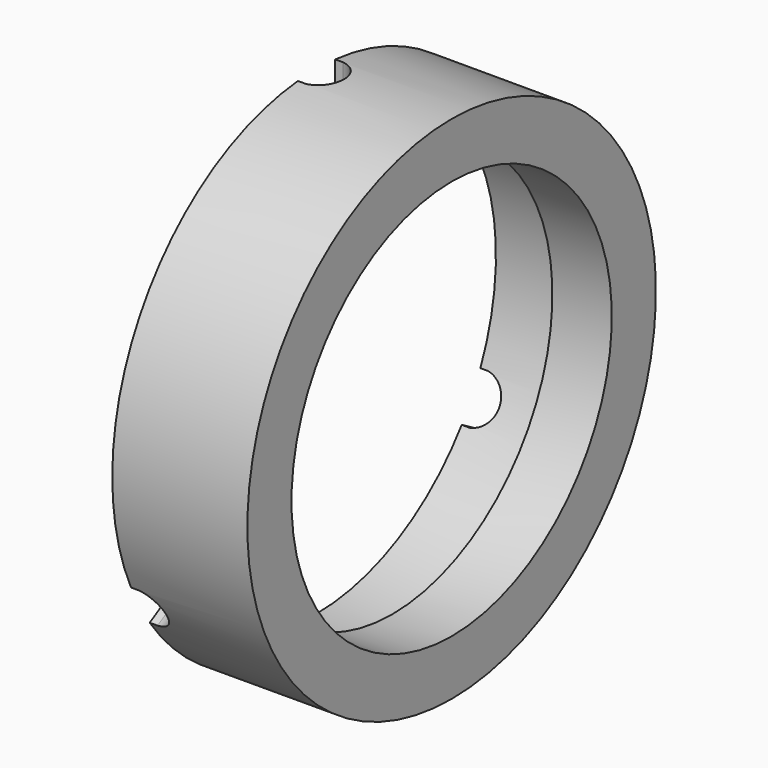
from build123d import *

# Parameters (mm, degrees)
F3_DEPTH        = 73.66
F3_COPIES_COUNT = 3
F4_R            = 0.4


# Not quite as in the source:
# - a pattern or mirror of a feature is missing from the dataset's text; its kind, count and spacing are read off the source's solid


with BuildPart() as f1:
    # F0 (on Front) → F1 (revolve)
    with BuildSketch(Plane.XZ):
        Polygon((28.7253968418, 54.2925000191), (0, 54.2925000191), (0, 47.6751327515), (16.0922370851, 47.6751327515), (16.0922370851, 42.5617098808), (28.7253968418, 42.5617098808), align=None)
    revolve(axis=Axis((14.3626984209, 0, 0), (1, 0, 0)))

    # F2 (on Top) → F3 (cut)
    with BuildSketch(Plane.XY):
        with BuildLine():
            Line((1.6697708597, 4.963026382), (0, 4.963026382))
            Line((0, 4.963026382), (-7.0685544051, 4.963026382))
            Line((-7.0685544051, 4.963026382), (-7.0685544051, -4.963026382))
            Line((-7.0685544051, -4.963026382), (0, -4.963026382))
            Line((0, -4.963026382), (1.6697708597, -4.963026382))
            ThreePointArc((1.6697708597, -4.963026382), (5.8676445687, 0), (1.6697708597, 4.963026382))
        make_face()
    f3 = extrude(amount=F3_DEPTH, mode=Mode.SUBTRACT)

    # F3_copies: F3 ×3 about axis
    f3_copies_axis = Axis((0, 0, 0), (1, 0, 0))
    for i in range(1, F3_COPIES_COUNT):
        add(f3.rotate(f3_copies_axis, i * 360 / F3_COPIES_COUNT), mode=Mode.SUBTRACT)

    # F4
    f4_edges = [f1.edges().sort_by_distance(p)[0] for p in [
        (16.092237, 0, -47.675133),
    ]]
    fillet(f4_edges, radius=F4_R)


solid = f1.part
